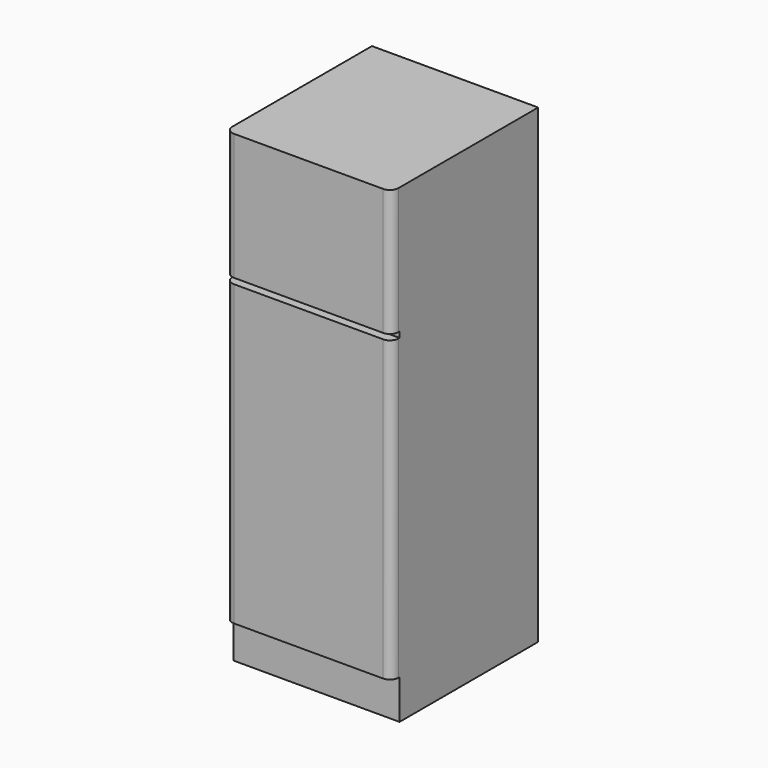
from build123d import *

# Parameters (mm, degrees)
F1_W     = 590
F1_H     = 650
F2_DEPTH = 1670
F3_W     = 35
F3_H     = 140
F3_H_2   = 20
F4_DEPTH = 590.001
F5_R     = 30


with BuildPart() as f2:
    # F1 (on Top) → F2 (new body)
    with BuildSketch(Plane.XY):
        with Locations((295, 325)):
            Rectangle(F1_W, F1_H)
    extrude(amount=F2_DEPTH)

    # F3 (on face) → F4 (cut, through all)
    with BuildSketch(Plane.YZ.offset(590)):
        with Locations((17.5, 70)):
            Rectangle(F3_W, F3_H)
        with Locations((17.5, 1210)):
            Rectangle(F3_W, F3_H_2)
    extrude(amount=-F4_DEPTH, mode=Mode.SUBTRACT)

    # F5
    f5_edges = [f2.edges().sort_by_distance(p)[0] for p in [
        (0, 0, 1445),
        (0, 0, 670),
        (590, 0, 670),
        (590, 0, 1445),
    ]]
    fillet(f5_edges, radius=F5_R)


solid = f2.part
